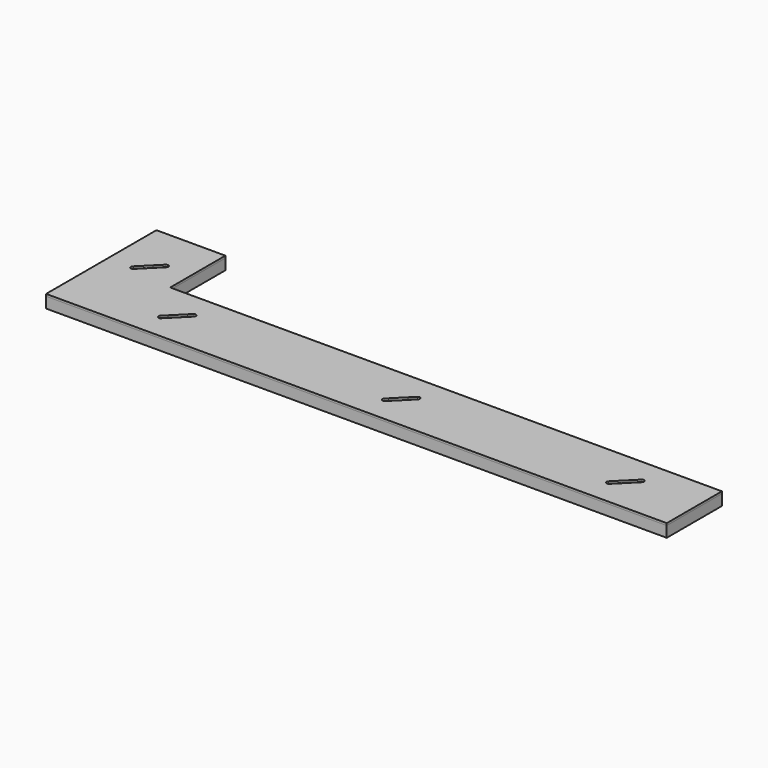
from build123d import *

# Parameters (mm, degrees)
F2_DEPTH = 19.05
F0_R     = 5.207
F3_DEPTH = 15.875


# Not quite as in the source:
# - a length typed as a fraction of an inch, garbled in the dataset ("3 / 203.2 mm" for 3/8 in), is restored


with BuildPart() as f2:
    # F1 (on face) → F2 (new body)
    with BuildSketch(Plane.XY):
        Polygon((101.6, 203.2), (0, 203.2), (0, 0), (914.4, 0), (914.4, 101.6), (101.6, 101.6), align=None)
        with BuildLine():
            Line((168.2052507731, 61.9355175901), (141.2644824099, 34.9947492269))
            ThreePointArc((141.2644824099, 34.9947492269), (136.5947492269, 34.9947492269), (136.5947492269, 39.6644824099))
            Line((136.5947492269, 39.6644824099), (163.5355175901, 66.6052507731))
            ThreePointArc((163.5355175901, 66.6052507731), (168.2052507731, 66.6052507731), (168.2052507731, 61.9355175901))
        make_face(mode=Mode.SUBTRACT)
        with BuildLine():
            Line((498.4052507731, 61.9355175901), (471.4644824099, 34.9947492269))
            ThreePointArc((471.4644824099, 34.9947492269), (466.7947492269, 34.9947492269), (466.7947492269, 39.6644824099))
            Line((466.7947492269, 39.6644824099), (493.7355175901, 66.6052507731))
            ThreePointArc((493.7355175901, 66.6052507731), (498.4052507731, 66.6052507731), (498.4052507731, 61.9355175901))
        make_face(mode=Mode.SUBTRACT)
        with BuildLine():
            Line((828.6052507731, 61.9355175901), (801.6644824099, 34.9947492269))
            ThreePointArc((801.6644824099, 34.9947492269), (796.9947492269, 34.9947492269), (796.9947492269, 39.6644824099))
            Line((796.9947492269, 39.6644824099), (823.9355175901, 66.6052507731))
            ThreePointArc((823.9355175901, 66.6052507731), (828.6052507731, 66.6052507731), (828.6052507731, 61.9355175901))
        make_face(mode=Mode.SUBTRACT)
        with BuildLine():
            Line((66.6052507731, 138.1355175901), (39.6644824099, 111.1947492269))
            ThreePointArc((39.6644824099, 111.1947492269), (34.9947492269, 111.1947492269), (34.9947492269, 115.8644824099))
            Line((34.9947492269, 115.8644824099), (61.9355175901, 142.8052507731))
            ThreePointArc((61.9355175901, 142.8052507731), (66.6052507731, 142.8052507731), (66.6052507731, 138.1355175901))
        make_face(mode=Mode.SUBTRACT)
    extrude(amount=F2_DEPTH)


with BuildPart() as f3:
    # F0 (on Top) → F3 (new body)
    with BuildSketch(Plane.XY):
        Polygon((101.6, 203.2), (0, 203.2), (0, 0), (914.4, 0), (914.4, 101.6), (101.6, 101.6), align=None)
        with Locations((152.4, 50.8)):
            Circle(F0_R, mode=Mode.SUBTRACT)
        with Locations((482.6, 50.8)):
            Circle(F0_R, mode=Mode.SUBTRACT)
        with Locations((812.8, 50.8)):
            Circle(F0_R, mode=Mode.SUBTRACT)
        with Locations((50.8, 127)):
            Circle(F0_R, mode=Mode.SUBTRACT)
    extrude(amount=F3_DEPTH)


solid = Compound([f2.part, f3.part])
